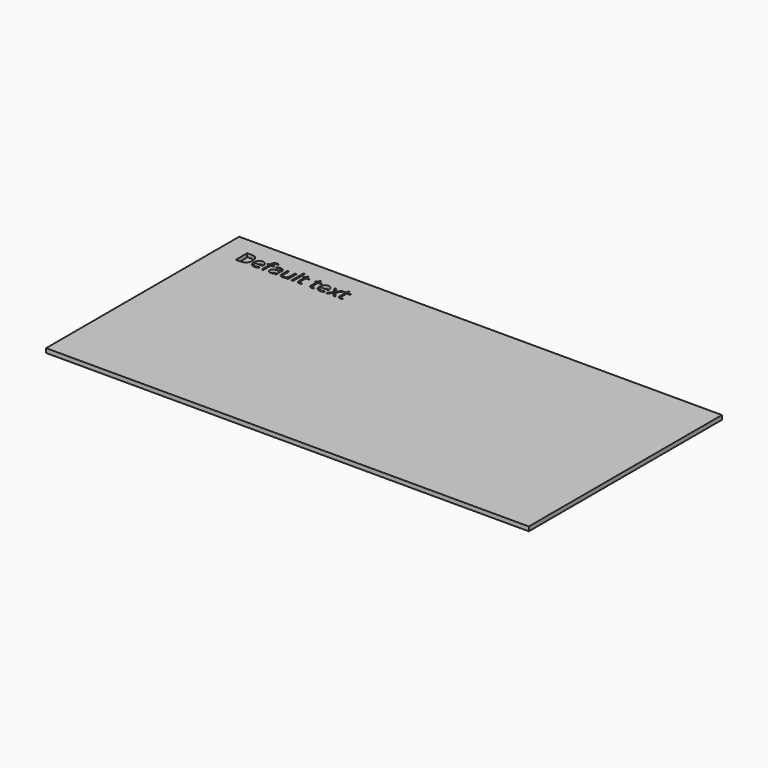
from build123d import *

# Parameters (mm, degrees)
F0_W         = 5080
F0_H         = 2540
F1_DEPTH     = 20
F2_TEXT_SIZE = 210.2583646774
F3_DEPTH     = 178
F4_DEPTH     = 25


# Not quite as in the source:
# - Text() gives the source's letters only with a copy of the font that has no kerning and outlines rounded to 1/6400 em; it was checked with that copy


with BuildPart() as f1:
    # F0 (on Top) → F1 (new body)
    with BuildSketch(Plane.XY):
        with Locations((2540, 1270)):
            Rectangle(F0_W, F0_H)
    extrude(amount=F1_DEPTH)

    # F2 (on face) → F3 (cut)
    with BuildSketch(Plane.XY.offset(20)):
        with Locations((214.1186147928, 2201.2090682983)):
            Text('Default text', F2_TEXT_SIZE, font='Open Sans', text_align=(TextAlign.LEFT, TextAlign.BOTTOM))
    extrude(amount=-F3_DEPTH, mode=Mode.SUBTRACT)

    # F4 (add): a face of the model
    f4_faces = [f1.faces().sort_by_distance(p)[0] for p in [
        (2548.7775351996, 1265.2627439193, 20),
    ]]
    extrude(f4_faces, amount=F4_DEPTH)


solid = f1.part
